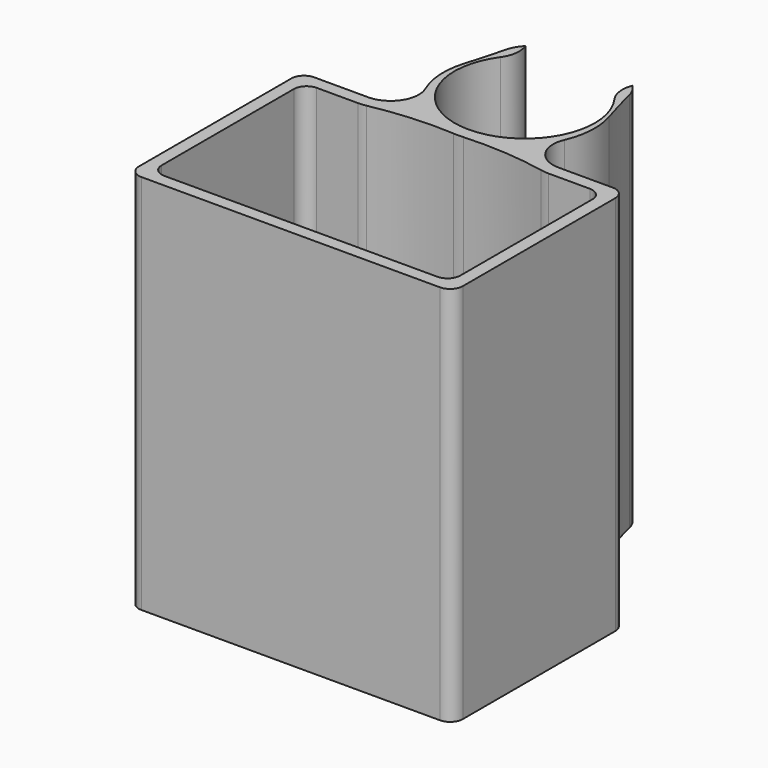
from build123d import *

# Parameters (mm, degrees)
F4_W        = 51
F4_H        = 32
F5_DEPTH    = 60
F6_T1_DEPTH = 60
F7_R        = 4.42
F9_T1_DEPTH = 77.3960297945
F10_T       = -2
F11_R       = 11
F12_DEPTH   = 2
F13_R       = 51
F14_R       = 2


# Not quite as in the source:
# - a fillet or chamfer that OpenCascade refuses, or shapes differently, is made with other operations: its cross-section is extruded or revolved along the edge and cut away or added
# - two fillets or chamfers of one size are made in one step


with BuildPart() as f5:
    # F4 (on Top) → F5 (new body)
    with BuildSketch(Plane.XY):
        with BuildLine():
            Line((-25.5, 0), (-25.5, -2))
            Line((-25.5, -2), (25.5, -2))
            Line((25.5, -2), (25.5, 0))
            Line((25.5, 0), (4.7777200824, 0))
            ThreePointArc((4.7777200824, 0), (0, -1), (-4.7777200824, 0))
            Line((-4.7777200824, 0), (-25.5, 0))
        make_face()
        with Locations((0, -18)):
            Rectangle(F4_W, F4_H)
        with BuildLine():
            ThreePointArc((-8.9084552032, 18.8231877912), (-11.6364061524, 8.3597035712), (-4.7777200824, 0))
            Line((-4.7777200824, 0), (4.7777200824, 0))
            ThreePointArc((4.7777200824, 0), (11.6364061524, 8.3597035712), (8.9084552032, 18.8231877912))
            ThreePointArc((8.9084552032, 18.8231877912), (8.2131677669, 19.5429454632), (7.4599259019, 20.2018099548))
            ThreePointArc((7.4599259019, 20.2018099548), (0, 1), (-7.4599259019, 20.2018099548))
            ThreePointArc((-7.4599259019, 20.2018099548), (-8.2131677669, 19.5429454632), (-8.9084552032, 18.8231877912))
        make_face()
        with BuildLine():
            Line((4.7777200824, 0), (-4.7777200824, 0))
            ThreePointArc((-4.7777200824, 0), (0, -1), (4.7777200824, 0))
        make_face()
        with BuildLine():
            Line((-8.9084552032, 23.9303167421), (-8.9084552032, 18.8231877912))
            ThreePointArc((-8.9084552032, 18.8231877912), (-8.2131677669, 19.5429454632), (-7.4599259019, 20.2018099548))
            Line((-7.4599259019, 20.2018099548), (-8.9084552032, 23.9303167421))
        make_face()
        with BuildLine():
            ThreePointArc((7.4599259019, 20.2018099548), (8.2131677669, 19.5429454632), (8.9084552032, 18.8231877912))
            Line((8.9084552032, 18.8231877912), (8.9084552032, 23.9303167421))
            Line((8.9084552032, 23.9303167421), (7.4599259019, 20.2018099548))
        make_face()
    extrude(amount=F5_DEPTH)

    # F6: fillet of radius 110.5 on 2 edges, made by hand

    # F6_s2 → F6_t1 (join)
    with BuildSketch(Plane.XY):
        with BuildLine():
            ThreePointArc((-8.9084552032, 23.9303167421), (-10.0405186332, 19.1502401697), (-11.3839102474, 14.4252006335))
            ThreePointArc((-11.3839102474, 14.4252006335), (-10.3817434304, 16.7567821247), (-8.9084552032, 18.8231877912))
            Line((-8.9084552032, 18.8231877912), (-8.9084552032, 23.9303167421))
        make_face()
        with BuildLine():
            ThreePointArc((11.3839102474, 14.4252006335), (10.0405186332, 19.1502401697), (8.9084552032, 23.9303167421))
            Line((8.9084552032, 23.9303167421), (8.9084552032, 18.8231877912))
            ThreePointArc((8.9084552032, 18.8231877912), (10.3817434304, 16.7567821247), (11.3839102474, 14.4252006335))
        make_face()
    extrude(amount=F6_T1_DEPTH)

    # F7
    f7_edges = [f5.edges().sort_by_distance(p)[0] for p in [
        (-4.77772, 0, 30),
        (4.77772, 0, 30),
        (7.459926, 20.20181, 30),
        (-7.459926, 20.20181, 30),
    ]]
    fillet(f7_edges, radius=F7_R)

    # F9: fillet of radius 4.42 on 2 edges, made by hand

    # F9_s2 → F9_t1 (cut)
    with BuildSketch(Plane.XY.offset(-8.6980148973)):
        with BuildLine():
            ThreePointArc((9.6882803435, 20.5396314345), (9.2143493926, 21.7090785299), (8.4292935977, 22.6969572949))
            Line((8.4292935977, 22.6969572949), (8.9084552032, 23.9303167421))
            ThreePointArc((8.9084552032, 23.9303167421), (9.2850220453, 22.2319046987), (9.6882803435, 20.5396314345))
        make_face()
        with BuildLine():
            ThreePointArc((-9.6882803435, 20.5396314345), (-9.2143493926, 21.7090785299), (-8.4292935977, 22.6969572949))
            Line((-8.4292935977, 22.6969572949), (-8.9084552032, 23.9303167421))
            ThreePointArc((-8.9084552032, 23.9303167421), (-9.2850220453, 22.2319046987), (-9.6882803435, 20.5396314345))
        make_face()
    extrude(amount=F9_T1_DEPTH, mode=Mode.SUBTRACT)

    # F10
    f10_openings = [f5.faces().sort_by_distance(p)[0] for p in [
        (0, -15.707049, 60),
    ]]
    offset(amount=F10_T, openings=f10_openings)

    # F11 (on face) → F12 (cut)
    with BuildSketch(Plane(origin=(0, 0, 0), x_dir=(1, 0, 0), z_dir=(0, 0, -1))):
        with Locations((7.5, 20)):
            Circle(F11_R)
    extrude(amount=-F12_DEPTH, mode=Mode.SUBTRACT)

    # F13
    f13_edges = [f5.edges().sort_by_distance(p)[0] for p in [
        (-8.868399, 2.47639, 31),
        (8.868399, 2.47639, 31),
    ]]
    fillet(f13_edges, radius=F13_R)

    # F14
    f14_edges = [f5.edges().sort_by_distance(p)[0] for p in [
        (-25.5, 0, 30),
        (25.5, 0, 30),
        (23.5, -32, 31),
        (-23.5, -32, 31),
        (25.5, -34, 30),
        (-25.5, -34, 30),
        (23.5, -2, 31),
        (-23.5, -2, 31),
    ]]
    fillet(f14_edges, radius=F14_R)


solid = f5.part
